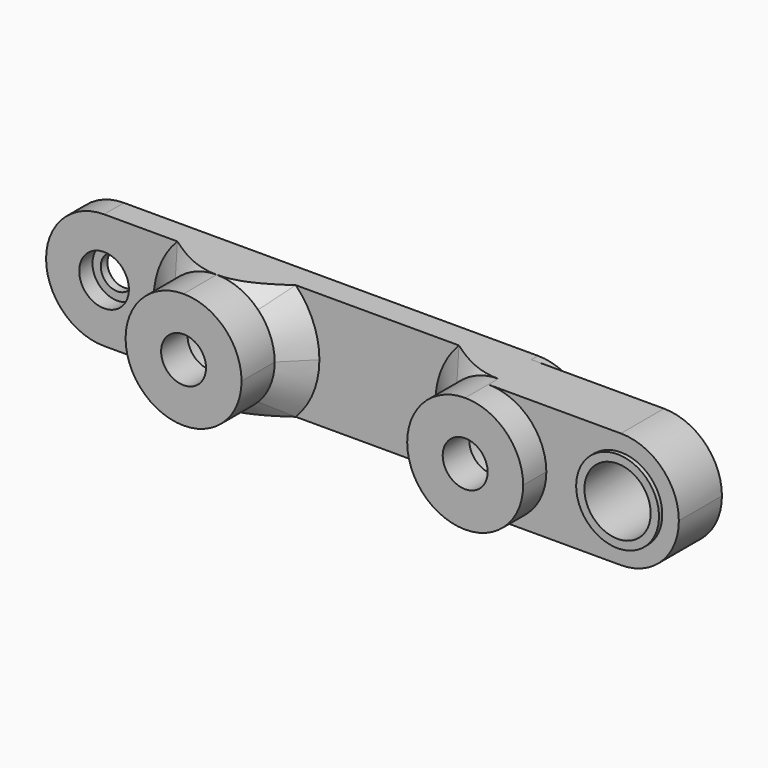
from build123d import *

# Parameters (mm, degrees)
F1_DEPTH      = 11.1125
F2_R          = 3.175
F2_R_2        = 1.5875
F2_R_3        = 2.15265
F3_DEPTH      = 8.73125
F4_R          = 2.38125
F5_DEPTH      = 1.5875
F6_R          = 3.96875
F6_R_2        = 3.175
F7_DEPTH      = 0.79375
F7_DEPTH_BACK = 5.55625
F8_R          = 5.55624
F10_R         = 3.96875
F11_DEPTH     = 5.55625
F12_C1_SIZE   = 2.38125
F12_C2_SIZE   = 2.38125
F12_C3_SIZE   = 2.38125


# Not quite as in the source:
# - a fillet or chamfer is up to 0.001 mm smaller than in the source, because OpenCascade refuses the exact size


with BuildPart() as f1:
    # F0 (on Top) → F1 (new body)
    with BuildSketch(Plane.XY):
        Polygon((-12.7, 0), (0, 0), (0, -6.35), (11.1125, -6.35), (11.1125, 0), (26.9875, 0), (26.9875, -6.35), (38.1, -6.35), (38.1, -3.571875), (50.8, -3.571875), (50.8, 1.5875), (38.1, 1.5875), (38.1, 2.38125), (-12.7, 2.38125), align=None)
    extrude(amount=F1_DEPTH)

    # F2 (on face) → F3 (cut, through all)
    with BuildSketch(Plane(origin=(0, 2.38125, 0), x_dir=(-1, 0, 0), z_dir=(0, 1, 0))):
        with Locations((-45.24375, 5.55625)):
            Circle(F2_R)
        with Locations((7.14375, 5.55625)):
            Circle(F2_R_2)
        with Locations((-5.55625, 5.55625)):
            Circle(F2_R_3)
        with Locations((-32.54375, 5.55625)):
            Circle(F2_R_3)
    extrude(amount=-F3_DEPTH, mode=Mode.SUBTRACT)

    # F4 (on face) → F5 (cut)
    with BuildSketch(Plane.XZ):
        with Locations((-7.14375, 5.55625)):
            Circle(F4_R)
    extrude(amount=-F5_DEPTH, mode=Mode.SUBTRACT)

    # F6 (on face) → F7 (join, two sides)
    with BuildSketch(Plane(origin=(0, 1.5875, 0), x_dir=(-1, 0, 0), z_dir=(0, 1, 0))) as f7_sk:
        with Locations((-45.24375, 5.55625)):
            Circle(F6_R)
        with Locations((-45.24375, 5.55625)):
            Circle(F6_R_2, mode=Mode.SUBTRACT)
    extrude(amount=F7_DEPTH)
    extrude(f7_sk.sketch, amount=-F7_DEPTH_BACK)

    # F8 (radius 5.55625 in the source; OpenCascade refuses exactly that, so slightly less here)
    f8_edges = [f1.edges().sort_by_distance(p)[0] for p in [
        (0, -3.175, 0),
        (0, -3.175, 11.1125),
        (38.1, -4.960938, 0),
        (38.1, -4.960938, 11.1125),
        (38.1, 1.984375, 0),
        (38.1, 1.984375, 11.1125),
        (11.1125, -3.175, 11.1125),
        (11.1125, -3.175, 0),
        (26.9875, -3.175, 11.1125),
        (26.9875, -3.175, 0),
        (50.8, -0.992188, 11.1125),
        (50.8, -0.992188, 0),
        (-12.7, 1.190625, 11.1125),
        (-12.7, 1.190625, 0),
    ]]
    fillet(f8_edges, radius=F8_R)

    # F10 (on face) → F11 (cut, through all)
    with BuildSketch(Plane(origin=(0, 2.38125, 0), x_dir=(-1, 0, 0), z_dir=(0, 1, 0))):
        with Locations((-32.54375, 5.55625)):
            Circle(F10_R)
        with Locations((-5.55625, 5.55625)):
            Circle(F10_R)
    extrude(amount=-F11_DEPTH, mode=Mode.SUBTRACT)

    # F12: chamfer of 2.38125 on 5 edges, made by hand

    # F12_c1
    f12_c1_edges = [f1.edges().sort_by_distance(p)[0] for p in [
        (1.6273850181, 0, 9.4851149819),
        (0, 0, 5.55625),
        (1.6273850181, 0, 1.6273850181),
    ]]
    chamfer(f12_c1_edges, length=F12_C1_SIZE)

    # F12_c2
    f12_c2_edges = [f1.edges().sort_by_distance(p)[0] for p in [
        (28.6148850181, 0, 9.4851149819),
        (26.9875, 0, 5.55625),
        (28.6148850181, 0, 1.6273850181),
    ]]
    chamfer(f12_c2_edges, length=F12_C2_SIZE)

    # F12_c3
    f12_c3_edges = [f1.edges().sort_by_distance(p)[0] for p in [
        (11.1125, 0, 5.55625),
        (9.4851149819, 0, 9.4851149819),
        (9.4851149819, 0, 1.6273850181),
    ]]
    chamfer(f12_c3_edges, length=F12_C3_SIZE)


solid = f1.part
